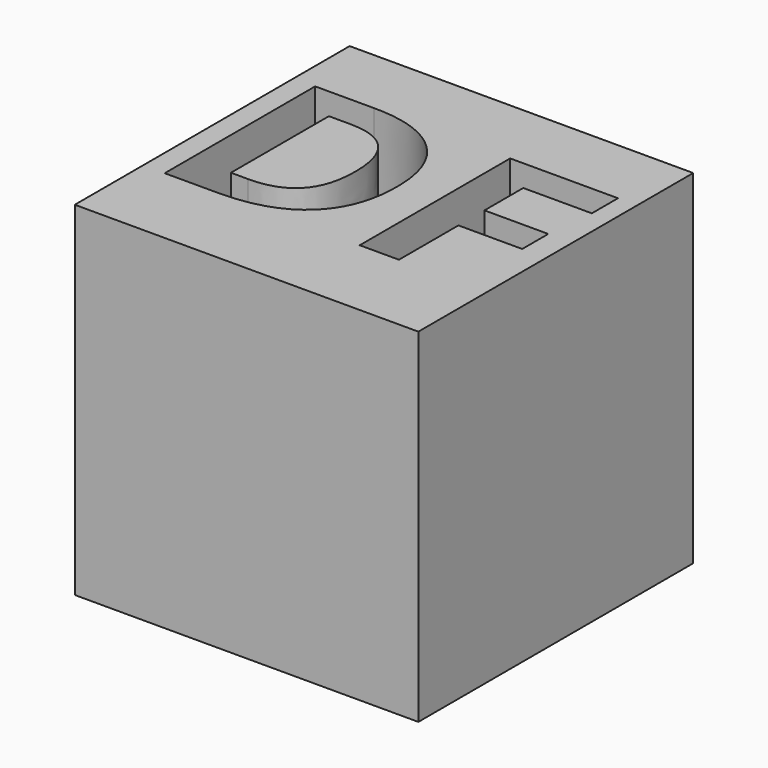
from build123d import *

# Parameters (mm, degrees)
F0_W         = 25.4
F0_H         = 25.4
F1_DEPTH     = 25.4
F2_TEXT_SIZE = 19.4752605727
F3_DEPTH     = 8.382
F4_TEXT_SIZE = 16.8020671835
F5_DEPTH     = 8.382


# Not quite as in the source:
# - Text() gives the source's letters only with a copy of the font that has no kerning and outlines rounded to 1/6400 em; it was checked with that copy


with BuildPart() as f1:
    # F0 (on Top) → F1 (new body)
    with BuildSketch(Plane.XY):
        with Locations((-0.9075403214, -0.1227975289)):
            Rectangle(F0_W, F0_H)
    extrude(amount=F1_DEPTH)

    # F2 (on face) → F3 (cut)
    with BuildSketch(Plane.XY.offset(25.4)):
        with Locations((-13.7668, -6.5024)):
            Text('DF', F2_TEXT_SIZE, font='Open Sans', font_style=FontStyle.BOLD, text_align=(TextAlign.LEFT, TextAlign.BOTTOM))
    extrude(amount=-F3_DEPTH, mode=Mode.SUBTRACT)

    # F4 (on face) → F5 (cut)
    with BuildSketch(Plane(origin=(0, 0, 0), x_dir=(1, 0, 0), z_dir=(0, 0, -1))):
        with Locations((-13.4991833078, -5.9184889231)):
            Text('DQ', F4_TEXT_SIZE, font='Open Sans', text_align=(TextAlign.LEFT, TextAlign.BOTTOM))
    extrude(amount=-F5_DEPTH, mode=Mode.SUBTRACT)


solid = f1.part
